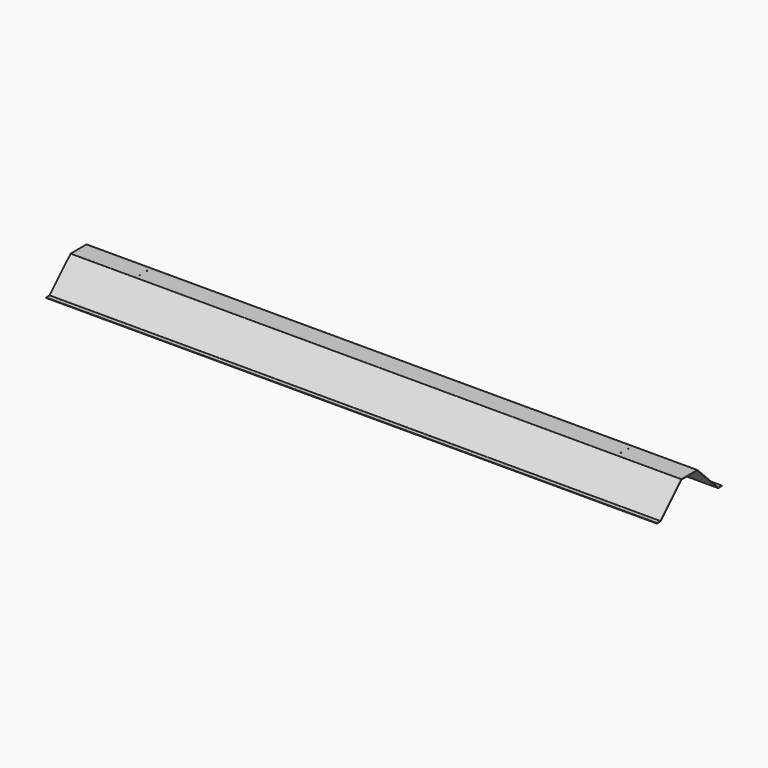
from build123d import *

# Parameters (mm, degrees)
F1_DEPTH = 1676.4
F3_R     = 3.175
F4_R     = 3.175
F6_D     = 5.1054


with BuildPart() as f1:
    # F0 (on Right) → F1 (new body, symmetric)
    with BuildSketch(Plane.YZ):
        Polygon((198.6212466711, 2.3228325226), (64.5779461899, 136.3661330038), (62.9354555616, 134.7236423755), (197.6590979371, 0), (223.0590979371, 0), (223.0590979371, 2.3228325226), align=None)
        Polygon((54.937148734, 146.0069304597), (0, 146.0069304597), (0, 143.6840979371), (53.975, 143.6840979371), (62.9354555616, 134.7236423755), (64.5779461899, 136.3661330038), align=None)
    extrude(amount=F1_DEPTH, both=True)

    # F2: F1 across face


with BuildPart() as f1_1:
    add(f1.part)
    add(f1.part.mirror(Plane(origin=(0, 0, 144.8455141984), x_dir=(1, 0, 0), z_dir=(0, -1, 0))))

    # F3
    f3_edges = [f1_1.edges().sort_by_distance(p)[0] for p in [
        (0, -54.937149, 146.00693),
        (0, -198.621247, 2.322833),
        (0, 54.937149, 146.00693),
        (0, 198.621247, 2.322833),
        (0, -197.659098, 0),
        (0, 197.659098, 0),
    ]]
    fillet(f3_edges, radius=F3_R)

    # F4
    f4_edges = [f1_1.edges().sort_by_distance(p)[0] for p in [
        (0, -53.975, 143.684098),
        (0, 53.975, 143.684098),
    ]]
    fillet(f4_edges, radius=F4_R)

    # F6 (through all)
    with Locations(Plane.XY.offset(146.0069304597)):
        with Locations((-1320.8, 25.4), (-1320.8, -25.4), (1320.8, 25.4), (1320.8, -25.4)):
            Hole(F6_D / 2)


solid = f1_1.part
